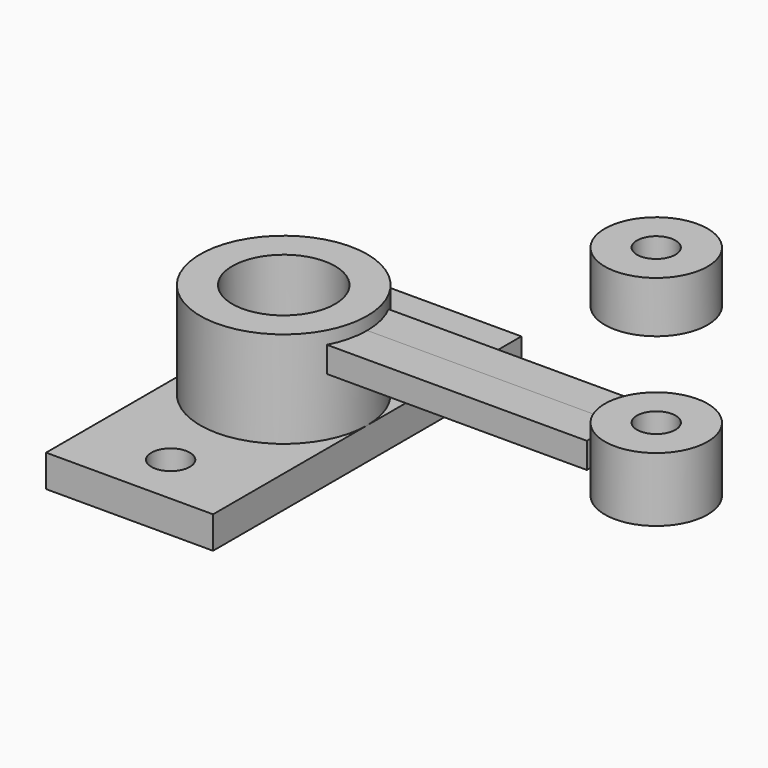
from build123d import *

# Parameters (mm, degrees)
F0_W      = 39
F0_H      = 90
F1_DEPTH  = 7.5
F3_R      = 4.5
F4_DEPTH  = 7.5
F5_DEPTH  = 22.5
F6_R      = 12
F7_DEPTH  = 30
F8_R      = 12
F9_DEPTH  = 15
F10_W     = 12
F10_H     = 12
F12_R     = 4.5
F13_DEPTH = 51
F14_R     = 4.5
F15_DEPTH = 15
F16_W     = 61
F16_H     = 6
F17_DEPTH = 9


with BuildPart() as f1:
    # F0 (on Top) → F1 (new body)
    with BuildSketch(Plane.XY):
        Rectangle(F0_W, F0_H)
    extrude(amount=F1_DEPTH)

    # F3 (on face) → F4 (cut, through all)
    with BuildSketch(Plane.XY.offset(7.5)):
        with Locations((0, -33)):
            Circle(F3_R)
        with Locations((0, 33)):
            Circle(F3_R)
    extrude(amount=-F4_DEPTH, mode=Mode.SUBTRACT)

    # F2 (on face) → F5 (join)
    with BuildSketch(Plane.XY.offset(7.5)):
        with BuildLine():
            ThreePointArc((-19.5, -2.3e-08), (1.15e-08, -19.5), (19.5, 0))
            ThreePointArc((19.5, 0), (-1.15e-08, 19.5), (-19.5, -2.3e-08))
        make_face()
    extrude(amount=F5_DEPTH)

    # F6 (on face) → F7 (cut, through all)
    with BuildSketch(Plane.XY.offset(30)):
        Circle(F6_R)
    extrude(amount=-F7_DEPTH, mode=Mode.SUBTRACT)

    # F14 (on face) → F15 (cut, through all)
    with BuildSketch(Plane.XY.offset(30)):
        with Locations((87, 0)):
            Circle(F14_R)
    extrude(amount=-F15_DEPTH, mode=Mode.SUBTRACT)


with BuildPart() as f9:
    # F8 (on face) → F9 (new body)
    with BuildSketch(Plane.XY.offset(30)):
        with Locations((87, 0)):
            Circle(F8_R)
    extrude(amount=-F9_DEPTH)


with BuildPart() as f11:
    # F10 (on Front) → F11 (revolve)
    with BuildSketch(Plane.XZ):
        with Locations((93, 60)):
            Rectangle(F10_W, F10_H)
    revolve(axis=Axis((87, 0, 60), (0, 0, -1)))


with BuildPart() as f13_tool:
    # F12 (on face) → F13 (new body, through all)
    with BuildSketch(Plane.XY.offset(66)):
        with Locations((87, 0)):
            Circle(F12_R)
    extrude(amount=-F13_DEPTH)


with BuildPart() as f9_1:
    add(f9.part)

    # F13: cut by f13_tool
    add(f13_tool.part, mode=Mode.SUBTRACT)


with BuildPart() as f11_1:
    add(f11.part)

    # F13: cut by f13_tool
    add(f13_tool.part, mode=Mode.SUBTRACT)


with BuildPart() as f17:
    # F16 (on Front) → F17 (new body)
    with BuildSketch(Plane.XZ):
        with Locations((47.5, 24)):
            Rectangle(F16_W, F16_H)
    extrude(amount=F17_DEPTH)


with BuildPart() as f18_1:
    # F18: instance of F17
    add(f17.part.mirror(Plane.XZ))


solid = Compound([f1.part, f9_1.part, f11_1.part, f17.part, f18_1.part])
